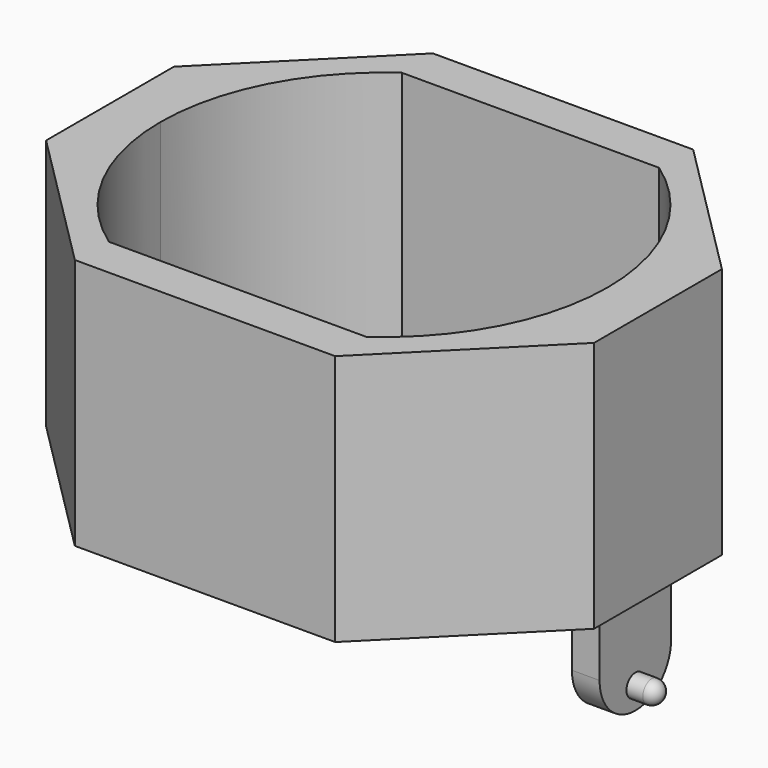
from build123d import *

# Parameters (mm, degrees)
F1_DEPTH  = 28.575
F3_DEPTH  = 6.35
F4_R      = 0.635
F5_DEPTH  = 1.5691231
F6_R      = 2.53999
F7_R      = 0.635
F9_DEPTH  = 6.35
F11_D     = 2.54
F16_D     = 127
F16_DEPTH = 20.6385


# Not quite as in the source:
# - a fillet or chamfer is up to 0.001 mm smaller than in the source, because OpenCascade refuses the exact size
# - a length typed as a fraction of an inch, garbled in the dataset ("3 / 203.2 mm" for 3/8 in), is restored
# - the program builds the solid bodies; features that only make, move or delete a surface that nothing else refers to are left out


with BuildPart() as f1:
    # F0 (on Top) → F1 (new body)
    with BuildSketch(Plane.XY):
        Polygon((7.3890909091, 12.7), (0, 12.7), (-7.3890909091, 12.7), (-15.5529601101, 4.536130799), (-15.5529601101, 0), (-15.5529601101, -4.536130799), (-7.3890909091, -12.7), (0, -12.7), (7.3890909091, -12.7), (15.5529601101, -4.536130799), (15.5529601101, 0), (15.5529601101, 4.536130799), align=None)
        with BuildLine():
            ThreePointArc((7.3019865971, 10.3909090909), (11.269987351, 5.8546891556), (12.7, 0))
            ThreePointArc((12.7, 0), (11.269987351, -5.8546891556), (7.3019865971, -10.3909090909))
            Line((7.3019865971, -10.3909090909), (0, -10.3909090909))
            Line((0, -10.3909090909), (-7.3019865971, -10.3909090909))
            ThreePointArc((-7.3019865971, -10.3909090909), (-11.269987351, -5.8546891556), (-12.7, 0))
            ThreePointArc((-12.7, 0), (-11.269987351, 5.8546891556), (-7.3019865971, 10.3909090909))
            Line((-7.3019865971, 10.3909090909), (0, 10.3909090909))
            Line((0, 10.3909090909), (7.3019865971, 10.3909090909))
        make_face(mode=Mode.SUBTRACT)
    extrude(amount=F1_DEPTH)

    # F2 (on Top) → F3 (join)
    with BuildSketch(Plane.XY):
        Polygon((14.2691231, -2.54), (14.2691231, 0), (14.2691231, 2.54), (12.7, 2.54), (12.7, 0), (12.7, -2.54), align=None)
    extrude(amount=-F3_DEPTH)

    # F4 (on face) → F5 (join)
    with BuildSketch(Plane.YZ.offset(14.2691231)):
        with Locations((0, -5.08)):
            Circle(F4_R)
    extrude(amount=F5_DEPTH)

    # F6 (radius 2.54 in the source; OpenCascade refuses exactly that, so slightly less here)
    f6_edges = [f1.edges().sort_by_distance(p)[0] for p in [
        (13.484562, -2.54, -6.35),
        (13.484562, 2.54, -6.35),
    ]]
    fillet(f6_edges, radius=F6_R)

    # F7
    f7_edges = [f1.edges().sort_by_distance(p)[0] for p in [
        (15.838246, -0.635, -5.08),
    ]]
    fillet(f7_edges, radius=F7_R)

    # F8 (on face) → F9 (join)
    with BuildSketch(Plane.XY.offset(28.575)):
        Polygon((15.5529601101, 2.54), (13.9838320495, 2.54), (13.9838320495, 0), (13.9838320495, -2.54), (15.5529601101, -2.54), (15.5529601101, 0), align=None)
    extrude(amount=F9_DEPTH)

    # F11 (through all)
    with Locations(Plane.YZ.offset(15.5529601101)):
        with Locations((0, 32.385)):
            Hole(F11_D / 2)

    # F12: F1 across plane


with BuildPart() as f1_1:
    add(f1.part)
    add(f1.part.mirror(Plane.YZ))

    # F16 (through all, one way)
    with BuildSketch(Plane(origin=(0, 0, 14.2875), x_dir=(1, 0, 0), z_dir=(0, 0, -1))):
        with Locations((0, 0)):
            Circle(F16_D / 2)
    extrude(amount=-F16_DEPTH, mode=Mode.SUBTRACT)


solid = f1_1.part
